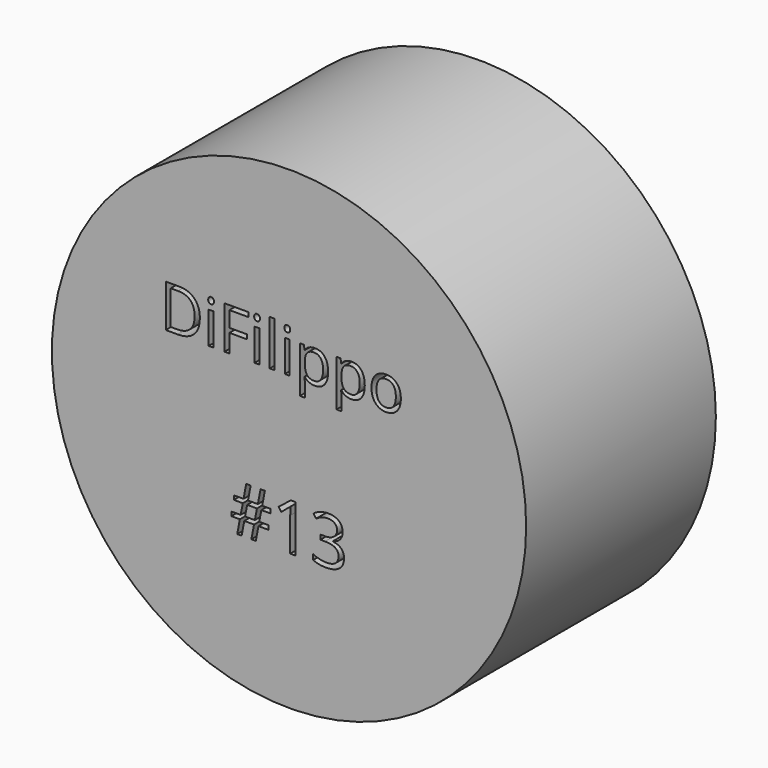
from build123d import *

# Parameters (mm, degrees)
F0_R         = 25.4
F1_DEPTH     = 25.4
F3_TEXT_SIZE = 7.0727462583
F4_DEPTH     = 25.4
F2_TEXT_SIZE = 6.4033626889
F5_DEPTH     = 25.4


# Not quite as in the source:
# - Text() gives the source's letters only with a copy of the font that has no kerning and outlines rounded to 1/6400 em; it was checked with that copy


with BuildPart() as f1:
    # F0 (on Front) → F1 (new body)
    with BuildSketch(Plane.XZ):
        with Locations((28.2388255, 15.8483199775)):
            Circle(F0_R)
    extrude(amount=F1_DEPTH)

    # F3 (on face) → F4 (cut)
    with BuildSketch(Plane.XZ.offset(25.4)):
        with Locations((21.8888255, 5.0529983839)):
            Text('#13', F3_TEXT_SIZE, font='Open Sans', text_align=(TextAlign.LEFT, TextAlign.BOTTOM))
    extrude(amount=-F4_DEPTH, mode=Mode.SUBTRACT)

    # F2 (on face) → F5 (cut)
    with BuildSketch(Plane.XZ.offset(25.4)):
        with Locations((14.4075639546, 21.8034461141)):
            Text('DiFilippo', F2_TEXT_SIZE, font='Open Sans', text_align=(TextAlign.LEFT, TextAlign.BOTTOM))
    extrude(amount=-F5_DEPTH, mode=Mode.SUBTRACT)


solid = f1.part
